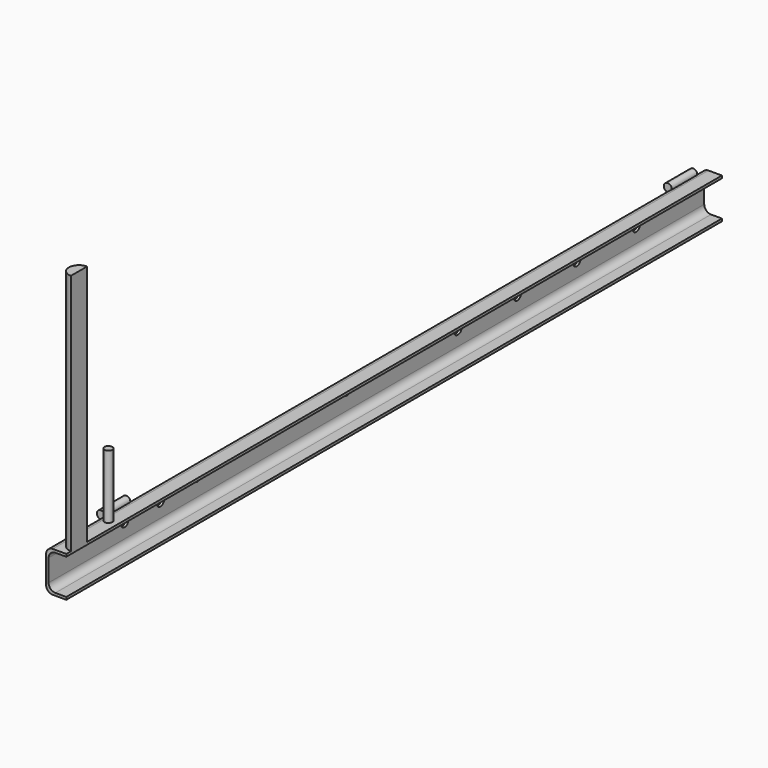
from build123d import *

# Parameters (mm, degrees)
F1_DEPTH  = 1525.228
F3_DEPTH  = 1525.228
F5_D      = 19
F5_DEPTH  = 5
F5_TIP    = 5.7081758808
F7_D      = 9
F7_DEPTH  = 5
F7_TIP    = 2.7038727856
F8_R      = 19.05
F9_DEPTH  = 457.2
F10_R     = 7.5
F11_DEPTH = 120
F12_DEPTH = 20
F16_R     = 7.5
F17_DEPTH = 60
F22_R     = 7.5
F23_DEPTH = 60
F28_D     = 15
F28_DEPTH = 5
F28_TIP   = 4.5064546427
F30_D     = 18
F30_DEPTH = 5
F30_TIP   = 5.4077455712
F32_D     = 10
F32_DEPTH = 5
F32_TIP   = 3.0043030951
F33_W     = 75
F33_H     = 1545.228
F34_DEPTH = 2500


# Not quite as in the source:
# - a feature names something its author has since deleted; it is built from what else it names


with BuildPart() as f1:
    # F0 (on Front) → F1 (new body)
    with BuildSketch(Plane.XZ):
        with BuildLine():
            ThreePointArc((0, 12.7), (3.7197438789, 3.7197438789), (12.7, 0))
            Line((12.7, 0), (63.5, 0))
            ThreePointArc((63.5, 0), (72.4802561211, 3.7197438789), (76.2, 12.7))
            Line((76.2, 12.7), (76.2, 63.5))
            ThreePointArc((76.2, 63.5), (72.4802561211, 72.4802561211), (63.5, 76.2))
            Line((63.5, 76.2), (12.7, 76.2))
            ThreePointArc((12.7, 76.2), (3.7197438789, 72.4802561211), (0, 63.5))
            Line((0, 63.5), (0, 12.7))
        make_face()
    extrude(amount=-F1_DEPTH)

    # F2 (on face) → F3 (cut)
    with BuildSketch(Plane.XZ):
        with BuildLine():
            Line((17.4625, 4.7625), (38.1, 4.7625))
            Line((38.1, 4.7625), (58.7375, 4.7625))
            ThreePointArc((58.7375, 4.7625), (67.7177561211, 8.4822438789), (71.4375, 17.4625))
            Line((71.4375, 17.4625), (71.4375, 58.7375))
            ThreePointArc((71.4375, 58.7375), (67.7177561211, 67.7177561211), (58.7375, 71.4375))
            Line((58.7375, 71.4375), (17.4625, 71.4375))
            ThreePointArc((17.4625, 71.4375), (8.4822438789, 67.7177561211), (4.7625, 58.7375))
            Line((4.7625, 58.7375), (4.7625, 17.4625))
            ThreePointArc((4.7625, 17.4625), (8.4822438789, 8.4822438789), (17.4625, 4.7625))
        make_face()
    extrude(amount=-F3_DEPTH, mode=Mode.SUBTRACT)

    # F5
    with Locations(Plane.YZ.offset(76.2)):
        with Locations((1335.228, 46.2), (1105.028, 46.2), (653.528, 46.2), (381.528, 46.2), (179.528, 46.2)):
            Hole(F5_D / 2, depth=F5_DEPTH)
            with Locations((0, 0, -(F5_DEPTH + F5_TIP / 2))):  # 118° drill point
                Cone(0, F5_D / 2, F5_TIP, mode=Mode.SUBTRACT)

    # F7
    with Locations(Plane.YZ.offset(76.2)):
        with Locations((261.933, 31.2), (501.133, 31.2), (760.333, 31.2), (979.533, 31.2), (1218.698, 31.2)):
            Hole(F7_D / 2, depth=F7_DEPTH)
            with Locations((0, 0, -(F7_DEPTH + F7_TIP / 2))):  # 118° drill point
                Cone(0, F7_D / 2, F7_TIP, mode=Mode.SUBTRACT)

    # F8 (on face) → F9 (join)
    with BuildSketch(Plane.XY.offset(76.2)):
        with Locations((38.1, 30)):
            Circle(F8_R)
    extrude(amount=F9_DEPTH)

    # F10 (on face) → F11 (join)
    with BuildSketch(Plane.XY.offset(76.2)):
        with Locations((20.2, 121.55)):
            Circle(F10_R)
    extrude(amount=F11_DEPTH)

    # F12 (add): a face of the model
    f12_faces = [f1.faces().sort_by_distance(p)[0] for p in [
        (1.0776307345, 1525.228, 38.1),
    ]]
    extrude(f12_faces, amount=F12_DEPTH)

    # F16 (on 3pt) → F17 (join)
    with BuildSketch(Plane.XZ.offset(-129.05)):
        with Locations((0, 76.2)):
            Circle(F16_R)
    extrude(amount=-F17_DEPTH)

    # F22 (on 3pt) → F23 (join)
    with BuildSketch(Plane(origin=(0, 1525.228, 0), x_dir=(-1, 0, 0), z_dir=(0, 1, 0))):
        with Locations((0, 76.2)):
            Circle(F22_R)
    extrude(amount=-F23_DEPTH)

    # F28
    with Locations(Plane.YZ.offset(76.2)):
        with Locations((1442.058, 31.2)):
            Hole(F28_D / 2, depth=F28_DEPTH)
            with Locations((0, 0, -(F28_DEPTH + F28_TIP / 2))):  # 118° drill point
                Cone(0, F28_D / 2, F28_TIP, mode=Mode.SUBTRACT)

    # F30
    with Locations(Plane(origin=(0, 0, 0), x_dir=(0, -1, 0), z_dir=(-1, 0, 0))):
        with Locations((-1385.03, 45.756), (-1244.831, 45.756), (-1104.633, 45.756), (-964.435, 45.756), (-263.443, 45.756), (-179.228, 45.756)):
            Hole(F30_D / 2, depth=F30_DEPTH)
            with Locations((0, 0, -(F30_DEPTH + F30_TIP / 2))):  # 118° drill point
                Cone(0, F30_D / 2, F30_TIP, mode=Mode.SUBTRACT)

    # F32
    with Locations(Plane(origin=(0, 0, 0), x_dir=(0, -1, 0), z_dir=(-1, 0, 0))):
        with Locations((-702.728, 47.406), (-350.228, 47.406)):
            Hole(F32_D / 2, depth=F32_DEPTH)
            with Locations((0, 0, -(F32_DEPTH + F32_TIP / 2))):  # 118° drill point
                Cone(0, F32_D / 2, F32_TIP, mode=Mode.SUBTRACT)

    # F33 (on face) → F34 (cut)
    with BuildSketch(Plane(origin=(0, 0, 0), x_dir=(1, 0, 0), z_dir=(0, 0, -1))):
        with Locations((75.6, -772.614)):
            Rectangle(F33_W, F33_H)
    extrude(amount=-F34_DEPTH, mode=Mode.SUBTRACT)


solid = f1.part
